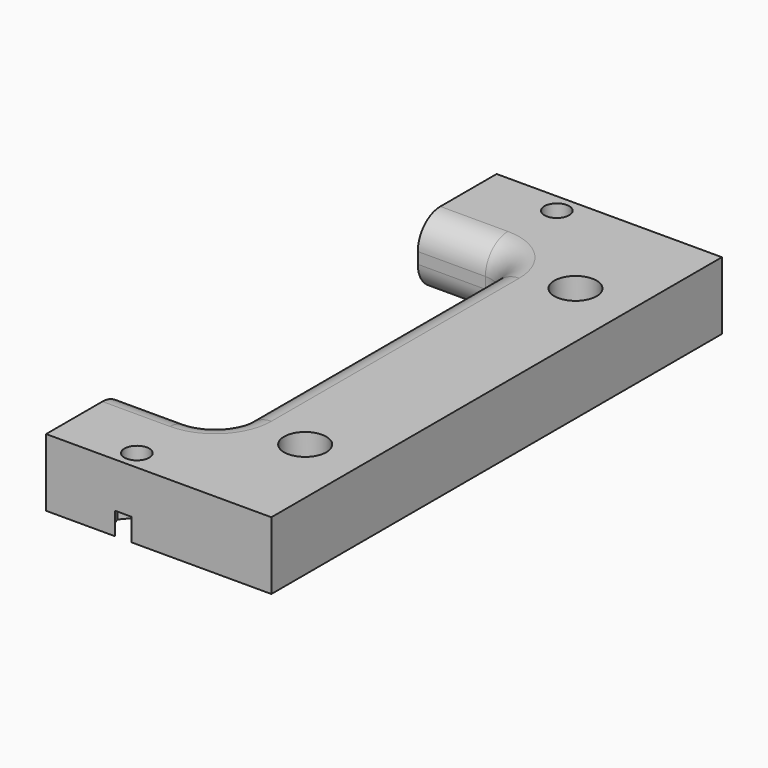
from build123d import *

# Parameters (mm, degrees)
F0_W     = 120
F0_H     = 100
F0_R     = 2.2
F1_DEPTH = 12
F2_R     = 3.75
F3_DEPTH = 5
F5_DEPTH = 4
F6_W     = 80
F6_H     = 100
F7_DEPTH = 25
F8_W     = 17
F8_H     = 65
F9_DEPTH = 25
F10_F1_R = 5
F10_F2_R = 5
F10_F3_R = 5


with BuildPart() as f1:
    # F0 (on Top) → F1 (new body)
    with BuildSketch(Plane.XY):
        Rectangle(F0_W, F0_H)
        with Locations((-46.6, -46.6)):
            Circle(F0_R, mode=Mode.SUBTRACT)
        with Locations((-30, -30)):
            Circle(F0_R, mode=Mode.SUBTRACT)
        with Locations((46.6, -46.6)):
            Circle(F0_R, mode=Mode.SUBTRACT)
        with Locations((30, -30)):
            Circle(F0_R, mode=Mode.SUBTRACT)
        with Locations((-46.6, 46.6)):
            Circle(F0_R, mode=Mode.SUBTRACT)
        with Locations((-30, 30)):
            Circle(F0_R, mode=Mode.SUBTRACT)
        with Locations((30, 30)):
            Circle(F0_R, mode=Mode.SUBTRACT)
        with Locations((46.6, 46.6)):
            Circle(F0_R, mode=Mode.SUBTRACT)
    extrude(amount=-F1_DEPTH)

    # F2 (on face) → F3 (cut)
    with BuildSketch(Plane.XY):
        with Locations((-30, 30)):
            Circle(F2_R)
        with Locations((30, 30)):
            Circle(F2_R)
        with Locations((30, -30)):
            Circle(F2_R)
        with Locations((-30, -30)):
            Circle(F2_R)
    extrude(amount=-F3_DEPTH, mode=Mode.SUBTRACT)

    # F4 (on face) → F5 (cut)
    with BuildSketch(Plane(origin=(0, 0, -12), x_dir=(1, 0, 0), z_dir=(0, 0, -1))):
        Polygon((-43.9383677783, 43.4813923112), (-42.5683904062, 47.3457372751), (-45.2300226279, 50.4643449639), (-49.2616322217, 49.7186076888), (-50.6316095938, 45.8542627249), (-47.9699773721, 42.7356550361), align=None)
        Polygon((46.3647294593, 42.5067558376), (50.0272181581, 44.3496276538), (50.2624886989, 48.4428718162), (46.8352705407, 50.6932441624), (43.1727818419, 48.8503723462), (42.9375113011, 44.7571281838), align=None)
        Polygon((-42.702877562, -45.3262509262), (-45.754537837, -42.5881184301), (-49.651660275, -43.8618675039), (-50.497122438, -47.8737490738), (-47.445462163, -50.6118815699), (-43.548339725, -49.3381324961), align=None)
        Polygon((50.5258183882, -45.4176506509), (47.5389646216, -42.6089668707), (43.6131462335, -43.7913162197), (42.6741816118, -47.7823493491), (45.6610353784, -50.5910331293), (49.5868537665, -49.4086837803), align=None)
    extrude(amount=-F5_DEPTH, mode=Mode.SUBTRACT)

    # F6 (on face) → F7 (cut)
    with BuildSketch(Plane.XY):
        with Locations((20, 0)):
            Rectangle(F6_W, F6_H)
    extrude(amount=-F7_DEPTH, mode=Mode.SUBTRACT)

    # F8 (on face) → F9 (cut)
    with BuildSketch(Plane.XY):
        with Locations((-51.5, 0)):
            Rectangle(F8_W, F8_H)
    extrude(amount=-F9_DEPTH, mode=Mode.SUBTRACT)

    # F10: fillet of radius 5 on 5 edges, made by hand

    # F10_f1
    f10_f1_edges = [f1.edges().sort_by_distance(p)[0] for p in [
        (-43, 32.5, -6),
        (-43, -32.5, -6),
    ]]
    fillet(f10_f1_edges, radius=F10_F1_R)

    # F10_f2
    f10_f2_edges = [f1.edges().sort_by_distance(p)[0] for p in [
        (-43, 0, -12),
        (-44.4644660941, -31.0355339059, -12),
        (-44.4644660941, 31.0355339059, -12),
    ]]
    fillet(f10_f2_edges, radius=F10_F2_R)

    # F10_f3
    f10_f3_edges = [f1.edges().sort_by_distance(p)[0] for p in [
        (-54, 32.5, 0),
        (-43, 0, 0),
        (-44.4644660941, -31.0355339059, 0),
        (-44.4644660941, 31.0355339059, 0),
    ]]
    fillet(f10_f3_edges, radius=F10_F3_R)


solid = f1.part
